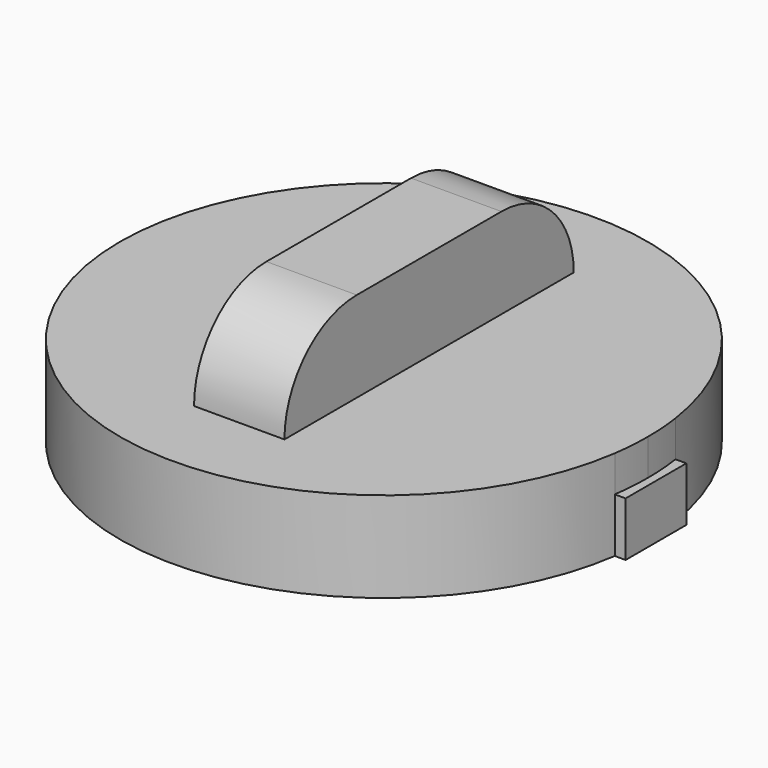
from build123d import *

# Parameters (mm, degrees)
F0_W     = 5
F0_H     = 20
F1_DEPTH = 5
F2_DEPTH = 3
F3_DEPTH = 10
F4_R     = 4.99999


# Not quite as in the source:
# - a fillet or chamfer is up to 0.001 mm smaller than in the source, because OpenCascade refuses the exact size


with BuildPart() as f1:
    # F0 (on Top) → F1 (new body)
    with BuildSketch(Plane.XY):
        with BuildLine():
            Line((14.4481832768, -2.1), (14.4481832768, 2.1))
            ThreePointArc((14.4481832768, 2.1), (0, 14.6), (-14.4481832768, 2.1))
            Line((-14.4481832768, 2.1), (-14.4037672862, 2.1))
            Line((-14.4037672862, 2.1), (-14.4037672862, -2.1))
            Line((-14.4037672862, -2.1), (-14.4481832768, -2.1))
            ThreePointArc((-14.4481832768, -2.1), (0, -14.6), (14.4481832768, -2.1))
        make_face()
        Rectangle(F0_W, F0_H, mode=Mode.SUBTRACT)
        with BuildLine():
            ThreePointArc((14.4481832768, -2.1), (14.5619963577, -1.0527402716), (14.6, 0))
            ThreePointArc((14.6, 0), (14.5619963577, 1.0527402716), (14.4481832768, 2.1))
            Line((14.4481832768, 2.1), (14.4481832768, -2.1))
        make_face()
        with BuildLine():
            Line((-14.4037672862, 2.1), (-14.4481832768, 2.1))
            ThreePointArc((-14.4481832768, 2.1), (-14.6, 0), (-14.4481832768, -2.1))
            Line((-14.4481832768, -2.1), (-14.4037672862, -2.1))
            Line((-14.4037672862, -2.1), (-14.4037672862, 2.1))
        make_face()
    extrude(amount=F1_DEPTH)

    # F0 (on Top) → F3 (join)
    with BuildSketch(Plane.XY):
        Rectangle(F0_W, F0_H)
    extrude(amount=F3_DEPTH)

    # F4 (radius 5 in the source; OpenCascade refuses exactly that, so slightly less here)
    f4_edges = [f1.edges().sort_by_distance(p)[0] for p in [
        (0, 10, 10),
        (0, -10, 10),
    ]]
    fillet(f4_edges, radius=F4_R)


with BuildPart() as f2:
    # F0 (on Top) → F2 (new body)
    with BuildSketch(Plane.XY):
        with BuildLine():
            ThreePointArc((-14.4481832768, -2.1), (-14.6, 0), (-14.4481832768, 2.1))
            Line((-14.4481832768, 2.1), (-15.0037672862, 2.1))
            Line((-15.0037672862, 2.1), (-15.0037672862, -2.1))
            Line((-15.0037672862, -2.1), (-14.4481832768, -2.1))
        make_face()
    extrude(amount=F2_DEPTH)


with BuildPart() as f2b:
    # F0 (on Top) → F2, piece 2 (new body)
    with BuildSketch(Plane.XY):
        with BuildLine():
            ThreePointArc((14.4481832768, 2.1), (14.5619963577, 1.0527402716), (14.6, 0))
            ThreePointArc((14.6, 0), (14.5619963577, -1.0527402716), (14.4481832768, -2.1))
            Line((14.4481832768, -2.1), (15.0481832768, -2.1))
            Line((15.0481832768, -2.1), (15.0481832768, 2.1))
            Line((15.0481832768, 2.1), (14.4481832768, 2.1))
        make_face()
    extrude(amount=F2_DEPTH)


solid = Compound([f1.part, f2.part, f2b.part])
